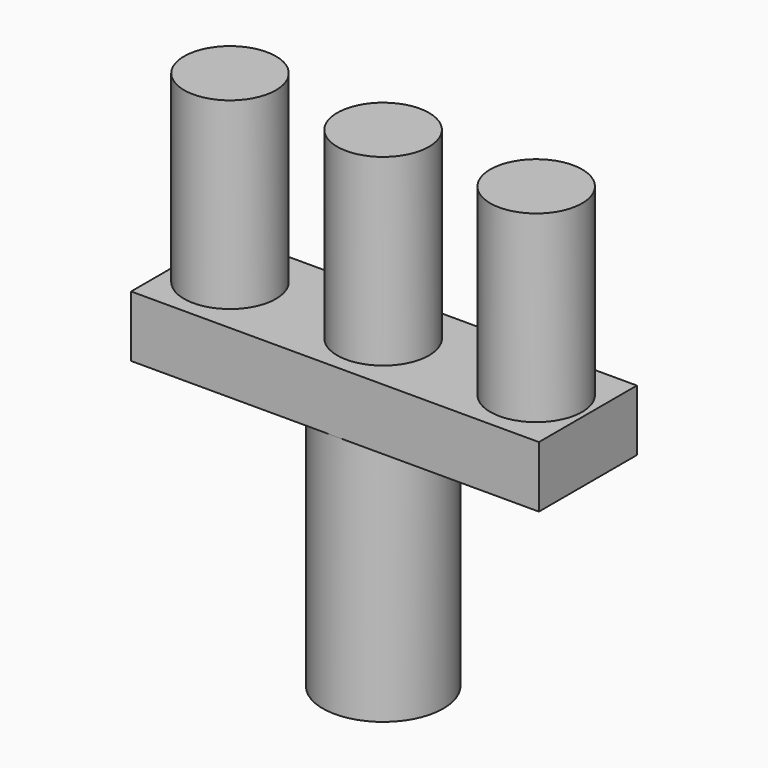
from build123d import *

# Parameters (mm, degrees)
F1_DEPTH = 40
F0_R     = 7.5
F0_W     = 66.5927492082
F0_H     = 20
F2_DEPTH = 10
F3_R     = 9.8529460541
F4_DEPTH = 40


with BuildPart() as f1:
    # F0 (on Top) → F1 (new body)
    with BuildSketch(Plane.XY):
        with BuildLine():
            ThreePointArc((-7.5, 0), (0, -7.5), (7.5, 0))
            ThreePointArc((7.5, 0), (0, 7.5), (-7.5, 0))
        make_face()
    extrude(amount=F1_DEPTH)


with BuildPart() as f1b:
    # F0 (on Top) → F1, piece 2 (new body)
    with BuildSketch(Plane.XY):
        with Locations((-25, 0)):
            Circle(F0_R)
    extrude(amount=F1_DEPTH)


with BuildPart() as f1c:
    # F0 (on Top) → F1, piece 3 (new body)
    with BuildSketch(Plane.XY):
        with BuildLine():
            ThreePointArc((32.5, 0), (25, 7.5), (17.5, 0))
            ThreePointArc((17.5, 0), (25, -7.5), (32.5, 0))
        make_face()
    extrude(amount=F1_DEPTH)


with BuildPart() as f2:
    # F0 (on Top) → F2 (new body)
    with BuildSketch(Plane.XY):
        with Locations((0.0907275826, 0.0664947927)):
            Rectangle(F0_W, F0_H)
        with Locations((-25, 0)):
            Circle(F0_R, mode=Mode.SUBTRACT)
        with BuildLine():
            ThreePointArc((-7.5, 0), (0, 7.5), (7.5, 0))
            ThreePointArc((7.5, 0), (0, -7.5), (-7.5, 0))
        make_face(mode=Mode.SUBTRACT)
        with BuildLine():
            ThreePointArc((32.5, 0), (25, -7.5), (17.5, 0))
            ThreePointArc((17.5, 0), (25, 7.5), (32.5, 0))
        make_face(mode=Mode.SUBTRACT)
    extrude(amount=F2_DEPTH)


with BuildPart() as f4:
    # F3 (on Top) → F4 (new body)
    with BuildSketch(Plane.XY):
        Circle(F3_R)
    extrude(amount=-F4_DEPTH)


solid = Compound([f1.part, f1b.part, f1c.part, f2.part, f4.part])
